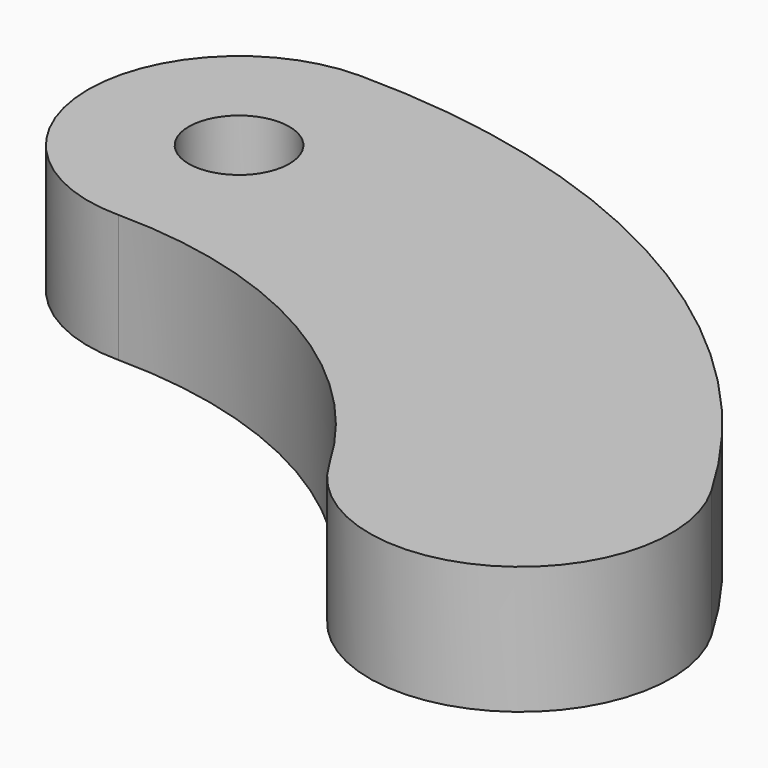
from build123d import *

# Parameters (mm, degrees)
F1_DEPTH = 6.35


# Not quite as in the source:
# - a length typed as a fraction of an inch, garbled in the dataset ("3 / 203.2 mm" for 3/8 in), is restored


with BuildPart() as f1:
    # F0 (on Top) → F1 (new body)
    with BuildSketch(Plane.XY):
        with BuildLine():
            ThreePointArc((0, 7.5), (-7.5, 0), (0, -7.5))
            ThreePointArc((0, -7.5), (11.25, -10.5144284149), (19.4855715851, -18.75))
            ThreePointArc((19.4855715851, -18.75), (29.7307621135, -21.4951905284), (32.4759526419, -11.25))
            ThreePointArc((32.4759526419, -11.25), (18.75, 2.4759526419), (0, 7.5))
        make_face()
        with BuildLine():
            ThreePointArc((2.4978289184, -0.1041666667), (-2.4994571707, 0.0520946447), (2.5, 0))
            ThreePointArc((2.5, 0), (2.4994571707, -0.0520946447), (2.4978289184, -0.1041666667))
        make_face(mode=Mode.SUBTRACT)
    extrude(amount=F1_DEPTH)


solid = f1.part
